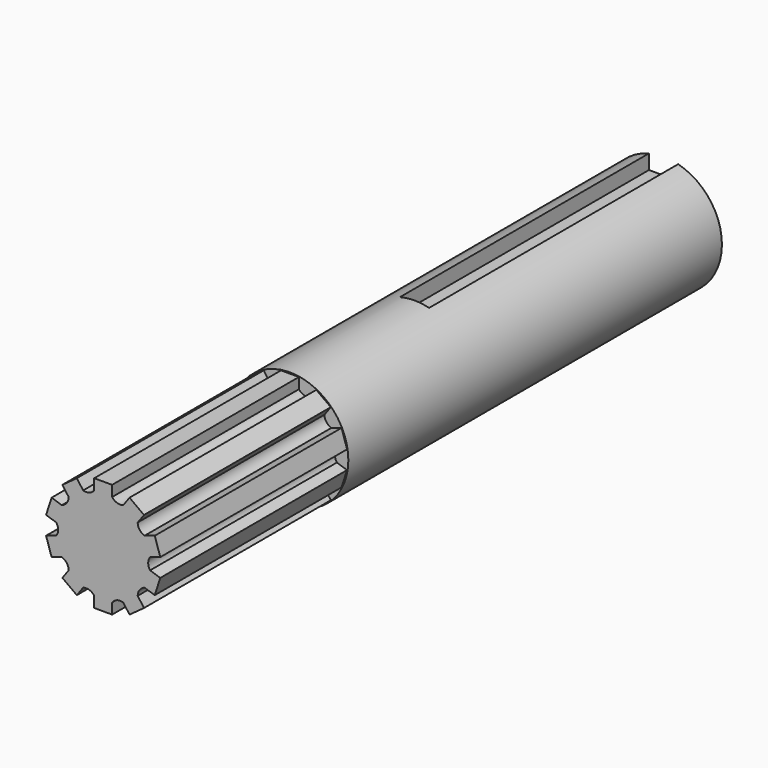
from build123d import *

# Parameters (mm, degrees)
F1_DEPTH = 38.1
F2_R     = 9.525
F3_DEPTH = 76.2
F5_DEPTH = 50.8


# Not quite as in the source:
# - a feature names something its author has since deleted; it is built from what else it names


with BuildPart() as f1:
    # F0 (on Front) → F1 (new body)
    with BuildSketch(Plane.XZ):
        with BuildLine():
            Line((1.4605, 7.5692852344), (1.4605, 9.3218852344))
            Line((1.4605, 9.3218852344), (-1.4605, 9.3218852344))
            Line((-1.4605, 9.3218852344), (-1.4605, 7.5692852344))
            ThreePointArc((-1.4605, 7.5692852344), (-2.2699762391, 6.9862685009), (-3.2675449109, 6.9821407509))
            Line((-3.2675449109, 6.9821407509), (-4.2976973441, 8.4000239352))
            Line((-4.2976973441, 8.4000239352), (-6.6608359846, 6.6831032133))
            Line((-6.6608359846, 6.6831032133), (-5.6306835515, 5.2652200289))
            ThreePointArc((-5.6306835515, 5.2652200289), (-5.9428749476, 4.3177513881), (-6.7474987256, 3.7280558148))
            Line((-6.7474987256, 3.7280558148), (-8.4143203761, 4.2696389991))
            Line((-8.4143203761, 4.2696389991), (-9.3169590166, 1.491602915))
            Line((-9.3169590166, 1.491602915), (-7.6501373662, 0.9500197307))
            ThreePointArc((-7.6501373662, 0.9500197307), (-7.3457974171, 0), (-7.6501373662, -0.9500197307))
            Line((-7.6501373662, -0.9500197307), (-9.3169590166, -1.491602915))
            Line((-9.3169590166, -1.491602915), (-8.4143203761, -4.2696389991))
            Line((-8.4143203761, -4.2696389991), (-6.7474987256, -3.7280558148))
            ThreePointArc((-6.7474987256, -3.7280558148), (-5.9428749476, -4.3177513881), (-5.6306835515, -5.2652200289))
            Line((-5.6306835515, -5.2652200289), (-6.6608359846, -6.6831032133))
            Line((-6.6608359846, -6.6831032133), (-4.2976973441, -8.4000239352))
            Line((-4.2976973441, -8.4000239352), (-3.2675449109, -6.9821407509))
            ThreePointArc((-3.2675449109, -6.9821407509), (-2.2699762391, -6.9862685009), (-1.4605, -7.5692852344))
            Line((-1.4605, -7.5692852344), (-1.4605, -9.3218852344))
            Line((-1.4605, -9.3218852344), (1.4605, -9.3218852344))
            Line((1.4605, -9.3218852344), (1.4605, -7.5692852344))
            ThreePointArc((1.4605, -7.5692852344), (2.2699762391, -6.9862685009), (3.2675449109, -6.9821407509))
            Line((3.2675449109, -6.9821407509), (4.2976973441, -8.4000239352))
            Line((4.2976973441, -8.4000239352), (6.6608359846, -6.6831032133))
            Line((6.6608359846, -6.6831032133), (5.6306835515, -5.2652200289))
            ThreePointArc((5.6306835515, -5.2652200289), (5.9428749476, -4.3177513881), (6.7474987256, -3.7280558148))
            Line((6.7474987256, -3.7280558148), (8.4143203761, -4.2696389991))
            Line((8.4143203761, -4.2696389991), (9.3169590166, -1.491602915))
            Line((9.3169590166, -1.491602915), (7.6501373662, -0.9500197307))
            ThreePointArc((7.6501373662, -0.9500197307), (7.3457974171, 0), (7.6501373662, 0.9500197307))
            Line((7.6501373662, 0.9500197307), (9.3169590166, 1.491602915))
            Line((9.3169590166, 1.491602915), (8.4143203761, 4.2696389991))
            Line((8.4143203761, 4.2696389991), (6.7474987256, 3.7280558148))
            ThreePointArc((6.7474987256, 3.7280558148), (5.9428749476, 4.3177513881), (5.6306835515, 5.2652200289))
            Line((5.6306835515, 5.2652200289), (6.6608359846, 6.6831032133))
            Line((6.6608359846, 6.6831032133), (4.2976973441, 8.4000239352))
            Line((4.2976973441, 8.4000239352), (3.2675449109, 6.9821407509))
            ThreePointArc((3.2675449109, 6.9821407509), (2.2699762391, 6.9862685009), (1.4605, 7.5692852344))
        make_face()
    extrude(amount=F1_DEPTH)

    # F2 (on Front) → F3 (join)
    with BuildSketch(Plane.XZ):
        Circle(F2_R)
    extrude(amount=-F3_DEPTH)

    # F4 (on face) → F5 (cut)
    with BuildSketch(Plane(origin=(0, 76.2, 0), x_dir=(-1, 0, 0), z_dir=(0, 1, 0))):
        with BuildLine():
            ThreePointArc((2.38125, 9.2225415932), (1.2001908859, 9.4490828569), (0, 9.525))
            ThreePointArc((0, 9.525), (-1.2001908859, 9.4490828569), (-2.38125, 9.2225415932))
            Line((-2.38125, 9.2225415932), (-2.38125, 6.8326))
            Line((-2.38125, 6.8326), (2.38125, 6.8326))
            Line((2.38125, 6.8326), (2.38125, 9.2225415932))
        make_face()
    extrude(amount=-F5_DEPTH, mode=Mode.SUBTRACT)


solid = f1.part
